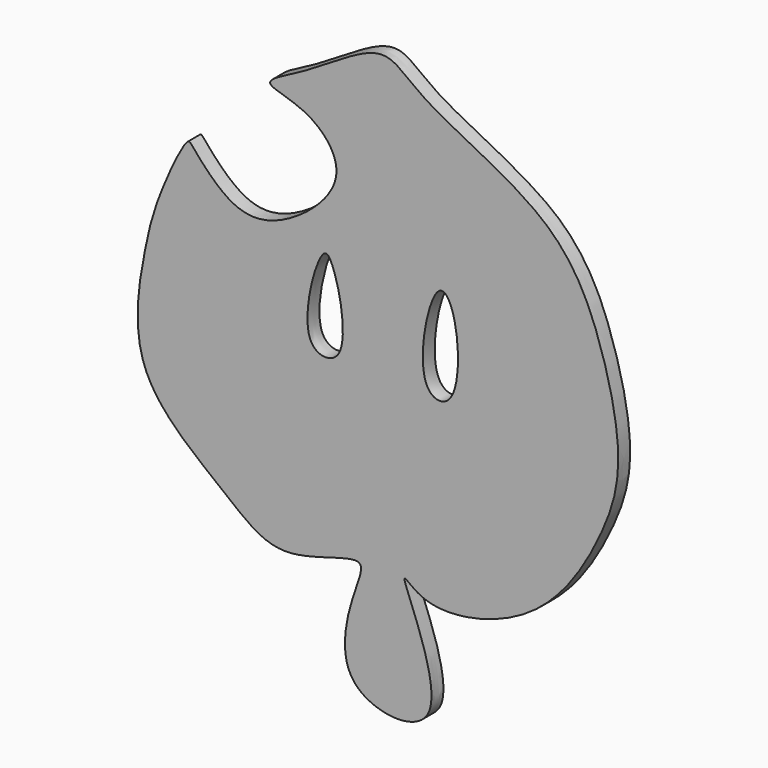
from build123d import *

# Parameters (mm, degrees)
F1_DEPTH = 2
F3_DEPTH = 25


with BuildPart() as f1:
    # F0 (on Front) → F1 (new body)
    with BuildSketch(Plane.XZ):
        with BuildLine():
            add(Edge.make_bspline(
                [(-57.0541098714, 56.5171316266), (-57.2866268412, 56.7940388881), (-57.8099420495, 57.3828138174), (-62.0118397294, 48.3290266809), (-63.3360182201, 42.4202077642), (-66.1876205351, 26.902784003), (-52.5736156709, 17.278329496), (-45.4489778331, 10.585401955), (-32.9990933315, 16.6025364294), (-35.7196893131, 10.3950428502), (-38.7543040419, -1.8875597472), (-19.5724357985, -3.8857429025), (-30.7652755168, 17.7600350203), (-25.5283502554, 11.3135430918), (-10.3681183128, 14.3261453392), (-2.1099477808, 27.8402459665), (1.0111687926, 37.5913378715), (-2.1521594771, 51.6778192577), (-8.3003787085, 64.298863189), (-26.4263176585, 71.2738417605), (-31.3926825349, 77.5705395748), (-40.6349636551, 70.3877473686), (-49.0806102, 66.9667253524), (-41.1671696619, 66.0423184361), (-35.2636128458, 59.2437252937), (-43.7000207578, 51.3298819182), (-51.4843082073, 49.7002297041), (-56.2266343763, 55.5316810871), (-57.0541098714, 56.5171316266)],
                knots=[0, 0, 0, 0, 0.0098628378, 0.0467661502, 0.0816760715, 0.1287785676, 0.178851731, 0.2183030326, 0.2577080229, 0.2825117159, 0.3244926909, 0.3640667088, 0.4133383704, 0.434501762, 0.4824975764, 0.5325673991, 0.5728277474, 0.6198687418, 0.6675009847, 0.722471933, 0.7544590924, 0.7966710721, 0.8279377522, 0.8562183097, 0.8906189754, 0.9298996506, 0.964900383, 1, 1, 1, 1], degree=3))
        make_face()
    extrude(amount=F1_DEPTH)

    # F2 (on face) → F3 (cut)
    with BuildSketch(Plane.XZ.offset(2)):
        with BuildLine():
            add(Edge.make_bspline(
                [(-39.3337756395, 49.5363920927), (-38.8999812076, 49.8268548099), (-37.9098480101, 48.0251074042), (-36.619318621, 42.8051228676), (-36.9612445875, 36.838702969), (-43.4637922782, 37.5726748153), (-40.496031852, 48.7581615007), (-39.3337756395, 49.5363920927)],
                knots=[0, 0, 0, 0, 0.1113941418, 0.3338555784, 0.534970773, 0.7015440406, 1, 1, 1, 1], degree=3))
        make_face()
        with BuildLine():
            add(Edge.make_bspline(
                [(-24.0298490971, 50.0733740628), (-23.3328350381, 50.631534343), (-21.2524507119, 47.9823976513), (-20.9813931291, 36.3407323094), (-27.699499266, 37.5494998073), (-25.4895464023, 48.9044664255), (-24.0298490971, 50.0733740628)],
                knots=[0, 0, 0, 0, 0.1625076552, 0.4852713722, 0.6596740291, 1, 1, 1, 1], degree=3))
        make_face()
    extrude(amount=-F3_DEPTH, mode=Mode.SUBTRACT)


solid = f1.part
